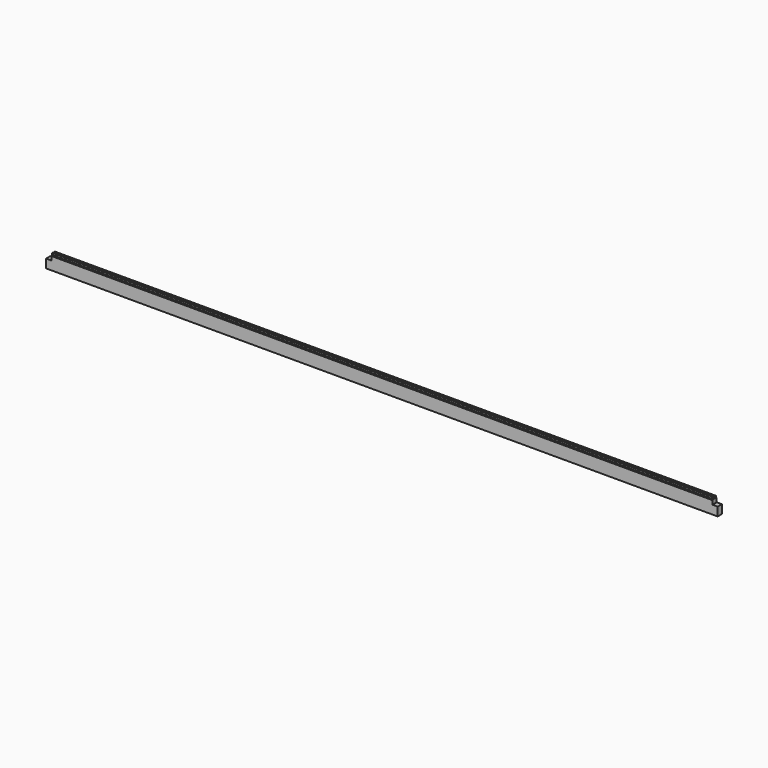
from build123d import *

# Parameters (mm, degrees)
F1_W     = 40
F1_H     = 33
F3_DEPTH = 2550
F2_W     = 80
F2_H     = 100
F4_DEPTH = 25
F5_W     = 5020
F5_H     = 19
F6_DEPTH = 40


with BuildPart() as f3:
    # F1 (on Right) → F3 (new body, symmetric)
    with BuildSketch(Plane.YZ):
        Polygon((20, 33), (20, 63), (17, 66), (12, 66), (12, 80), (4, 80), (4, 66), (-4, 66), (-4, 80), (-12, 80), (-12, 66), (-17, 66), (-20, 63), (-20, 33), align=None)
        with Locations((0, 16.5)):
            Rectangle(F1_W, F1_H)
        with Locations((0, -16.5)):
            Rectangle(F1_W, F1_H)
        Polygon((20, -52), (20, -33), (-20, -33), (-20, -52), (-12, -52), (-4, -52), (4, -52), (12, -52), align=None)
    extrude(amount=F3_DEPTH, both=True)

    # F2 (on Front) → F4 (cut, symmetric)
    with BuildSketch(Plane.XZ):
        with Locations((-2550, 83)):
            Rectangle(F2_W, F2_H)
        with Locations((-2550, -83)):
            Rectangle(F2_W, F2_H)
        with Locations((2550, 83)):
            Rectangle(F2_W, F2_H)
        with Locations((2550, -83)):
            Rectangle(F2_W, F2_H)
    extrude(amount=F4_DEPTH, both=True, mode=Mode.SUBTRACT)

    # F5 (on face) → F6 (cut, through all)
    with BuildSketch(Plane.XZ.offset(20)):
        with Locations((0, -42.5)):
            Rectangle(F5_W, F5_H)
    extrude(amount=-F6_DEPTH, mode=Mode.SUBTRACT)


solid = f3.part
